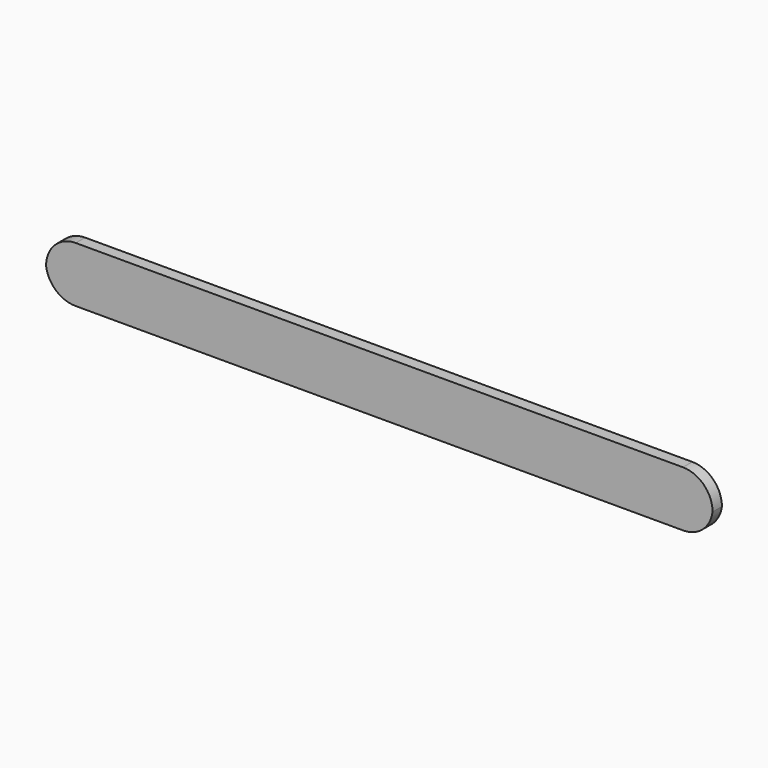
from build123d import *

# Parameters (mm, degrees)
F0_W        = 114.3
F0_H        = 9.525
F1_DEPTH    = 2.0066
F2_R        = 5.08
F3_T1_DEPTH = 27.2073812379
F4_R        = 5.08
F5_T1_DEPTH = 27.2073812379


# Not quite as in the source:
# - a fillet or chamfer that OpenCascade refuses, or shapes differently, is made with other operations: its cross-section is extruded or revolved along the edge and cut away or added


with BuildPart() as f1:
    # F0 (on Front) → F1 (new body)
    with BuildSketch(Plane.XZ):
        with Locations((-10.4238372296, -33.6832711485)):
            Rectangle(F0_W, F0_H)
    extrude(amount=F1_DEPTH)

    # F2
    f2_edges = [f1.edges().sort_by_distance(p)[0] for p in [
        (46.726163, -1.0033, -28.920771),
    ]]
    fillet(f2_edges, radius=F2_R)

    # F3: fillet of radius 5.08 on 1 edges, made by hand

    # F3_s2 → F3_t1 (cut)
    with BuildSketch(Plane.XZ.offset(-12.6003906189)):
        with BuildLine():
            ThreePointArc((46.7261627704, -34.0007711485), (45.0461106879, -37.1757711485), (41.6860065228, -38.4457711485))
            Line((41.6860065228, -38.4457711485), (46.7261627704, -38.4457711485))
            Line((46.7261627704, -38.4457711485), (46.7261627704, -34.0007711485))
        make_face()
    extrude(amount=F3_T1_DEPTH, mode=Mode.SUBTRACT)

    # F4
    f4_edges = [f1.edges().sort_by_distance(p)[0] for p in [
        (-67.573837, -1.0033, -28.920771),
    ]]
    fillet(f4_edges, radius=F4_R)

    # F5: fillet of radius 5.08 on 1 edges, made by hand

    # F5_s2 → F5_t1 (cut)
    with BuildSketch(Plane.XZ.offset(-12.6003906189)):
        with BuildLine():
            ThreePointArc((-67.5738372296, -34.0007711485), (-65.8937851471, -37.1757711485), (-62.533680982, -38.4457711485))
            Line((-62.533680982, -38.4457711485), (-67.5738372296, -38.4457711485))
            Line((-67.5738372296, -38.4457711485), (-67.5738372296, -34.0007711485))
        make_face()
    extrude(amount=F5_T1_DEPTH, mode=Mode.SUBTRACT)


solid = f1.part
